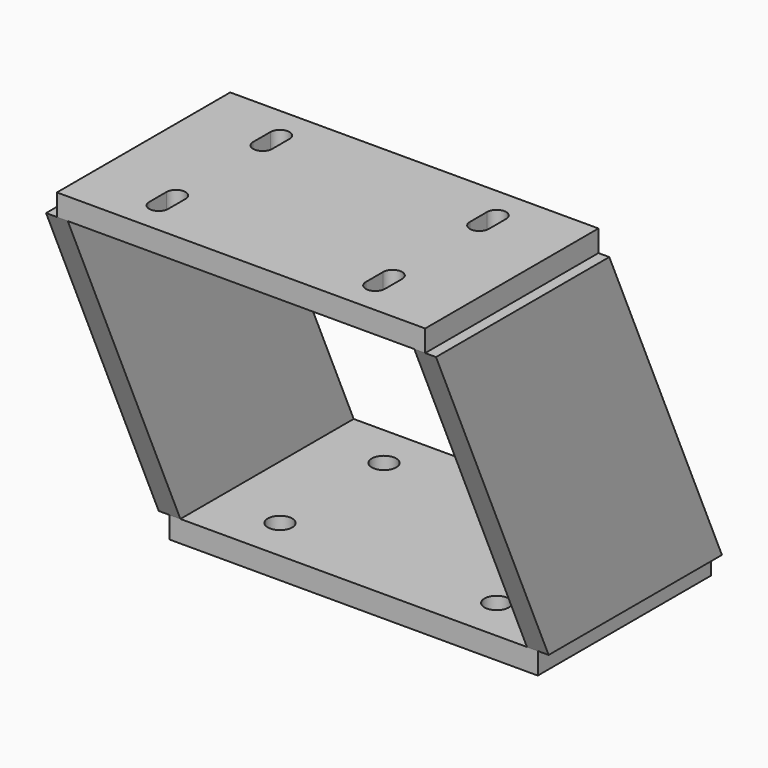
from build123d import *

# Parameters (mm, degrees)
F0_W      = 215.9
F0_H      = 127
F1_DEPTH  = 12.7
F3_D      = 14.2875
F5_W      = 215.9
F5_H      = 127
F6_DEPTH  = 12.7
F8_DEPTH  = 212.726
F10_DEPTH = 6.35


# Not quite as in the source:
# - a length typed as a fraction of an inch, garbled in the dataset ("3 / 203.2 mm" for 3/8 in), is restored


with BuildPart() as f1:
    # F0 (on Top) → F1 (new body)
    with BuildSketch(Plane.XY):
        Rectangle(F0_W, F0_H)
    extrude(amount=F1_DEPTH)

    # F3 (through all)
    with Locations(Plane.XY.offset(12.7)):
        with Locations((-63.5, 38.1), (63.5, 38.1), (63.5, -38.1), (-63.5, -38.1)):
            Hole(F3_D / 2)



with BuildPart() as f6:
    # F5 (on offset) → F6 (new body)
    with BuildSketch(Plane.XY.offset(212.725)):
        with Locations((0, -82.55)):
            Rectangle(F5_W, F5_H)
    extrude(amount=-F6_DEPTH)

    # F7 (on face) → F8 (cut, through all)
    with BuildSketch(Plane.XY.offset(212.725)):
        with BuildLine():
            ThreePointArc((-57.94375, -38.1), (-63.5, -32.54375), (-69.05625, -38.1))
            Line((-69.05625, -38.1), (-69.05625, -50.8))
            ThreePointArc((-69.05625, -50.8), (-63.5, -56.35625), (-57.94375, -50.8))
            Line((-57.94375, -50.8), (-57.94375, -38.1))
        make_face()
        with BuildLine():
            ThreePointArc((-57.94375, -114.3), (-63.5, -108.74375), (-69.05625, -114.3))
            Line((-69.05625, -114.3), (-69.05625, -127))
            ThreePointArc((-69.05625, -127), (-63.5, -132.55625), (-57.94375, -127))
            Line((-57.94375, -127), (-57.94375, -114.3))
        make_face()
        with BuildLine():
            ThreePointArc((69.05625, -38.1), (63.5, -32.54375), (57.94375, -38.1))
            Line((57.94375, -38.1), (57.94375, -50.8))
            ThreePointArc((57.94375, -50.8), (63.5, -56.35625), (69.05625, -50.8))
            Line((69.05625, -50.8), (69.05625, -38.1))
        make_face()
        with BuildLine():
            ThreePointArc((69.05625, -114.3), (63.5, -108.74375), (57.94375, -114.3))
            Line((57.94375, -114.3), (57.94375, -127))
            ThreePointArc((57.94375, -127), (63.5, -132.55625), (69.05625, -127))
            Line((69.05625, -127), (69.05625, -114.3))
        make_face()
    extrude(amount=-F8_DEPTH, mode=Mode.SUBTRACT)


with BuildPart() as f1_1:
    add(f1.part)

    add(f6.part)  # F10 merges F6
    # F9 (on face) → F10 (join, symmetric)
    with BuildSketch(Plane.YZ.offset(107.95)):
        Polygon((63.5, 12.7), (-19.05, 200.025), (-146.05, 200.025), (-63.5, 12.7), align=None)
    extrude(amount=F10_DEPTH, both=True)

    # F11: F1 across plane


with BuildPart() as f1_2:
    add(f1_1.part)
    add(f1_1.part.mirror(Plane.YZ))


solid = f1_2.part
